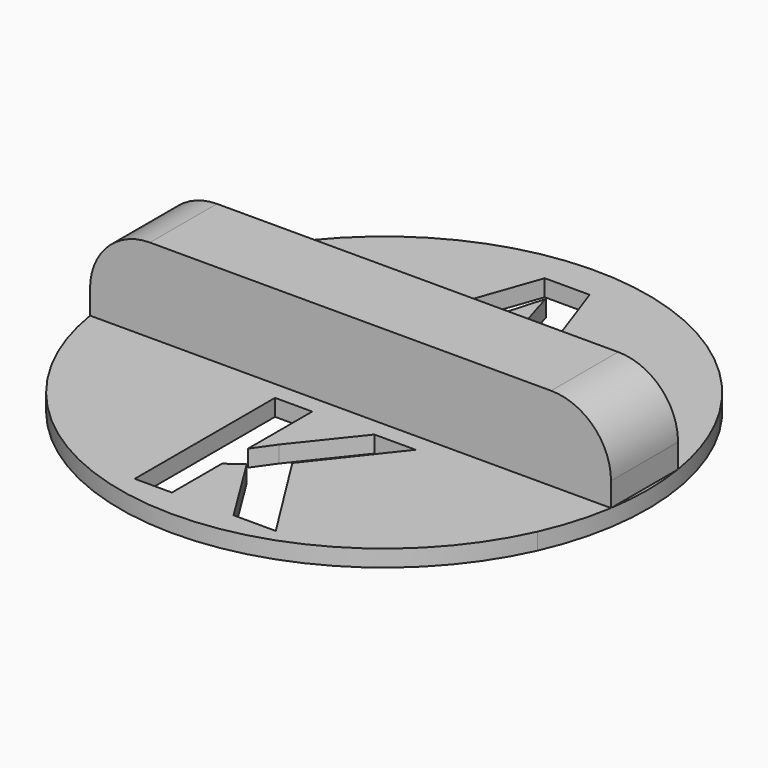
from build123d import *

# Parameters (mm, degrees)
F0_R          = 22.05
F1_DEPTH      = 1.4
F2_W          = 46.8786589982
F2_H          = 7
F3_DEPTH      = 7
F5_DEPTH      = 25
F7_DEPTH      = 25
F8_TEXT_SIZE  = 20.2705436904
F9_DEPTH      = 5
F10_TEXT_SIZE = 20.5177373977
F11_DEPTH     = 5


# Not quite as in the source:
# - Text() gives the source's letters only with a copy of the font that has no kerning and outlines rounded to 1/6400 em; it was checked with that copy


with BuildPart() as f1:
    # F0 (on Top) → F1 (new body)
    with BuildSketch(Plane.XY):
        Circle(F0_R)
    extrude(amount=F1_DEPTH)

    # F2 (on face) → F3 (join)
    with BuildSketch(Plane.XY.offset(1.4)):
        with Locations((0.6869044155, 0)):
            Rectangle(F2_W, F2_H)
    extrude(amount=F3_DEPTH)

    # F4 (on face) → F5 (cut)
    with BuildSketch(Plane.XY.offset(8.4)):
        with BuildLine():
            ThreePointArc((-20.2244413299, -8.784900278), (-22.0433329653, 0.1174414881), (-20.1296882775, 8.9998972133))
            Line((-20.1296882775, 8.9998972133), (-25.9023997933, 9.5238303766))
            Line((-25.9023997933, 9.5238303766), (-31.1410278082, -2.8289805632))
            Line((-31.1410278082, -2.8289805632), (-22.4099829793, -9.3610957265))
            Line((-22.4099829793, -9.3610957265), (-20.2244413299, -8.784900278))
        make_face()
        with BuildLine():
            Line((25.7077720016, 10.687969625), (18.850679885, 11.4391594041))
            ThreePointArc((18.850679885, 11.4391594041), (21.982729234, 1.3208352243), (20.0847610929, -9.0997182286))
            Line((20.0847610929, -9.0997182286), (27.3893084377, -8.0676069483))
            Line((27.3893084377, -8.0676069483), (31.0110747814, 2.2802972235))
            Line((31.0110747814, 2.2802972235), (25.7077720016, 10.687969625))
        make_face()
    extrude(amount=-F5_DEPTH, mode=Mode.SUBTRACT)

    # F6 (on face) → F7 (cut)
    with BuildSketch(Plane.XZ.offset(3.5)):
        with BuildLine():
            Line((-21.7650406008, 1.4), (-21.7650406008, 3.4))
            ThreePointArc((-21.7650406008, 3.4), (-20.3005745067, 6.9355339059), (-16.7650406008, 8.4))
            Line((-16.7650406008, 8.4), (-18.4185161579, 12.5083358405))
            Line((-18.4185161579, 12.5083358405), (-23.9234212786, 13.1551828235))
            Line((-23.9234212786, 13.1551828235), (-25.3046993166, 1.4))
            Line((-25.3046993166, 1.4), (-21.7650406008, 1.4))
        make_face()
        with BuildLine():
            ThreePointArc((16.7482826126, 8.4), (20.2838165185, 6.9355339059), (21.7482826126, 3.4))
            Line((21.7482826126, 3.4), (21.7482826126, 1.4))
            Line((21.7482826126, 1.4), (24.0328777581, 1.4))
            Line((24.0328777581, 1.4), (25.5436524749, 1.8891216023))
            Line((25.5436524749, 1.8891216023), (26.36378631, 8.6660245433))
            Line((26.36378631, 8.6660245433), (17.9466158152, 11.6875739768))
            Line((17.9466158152, 11.6875739768), (16.7482826126, 8.4))
        make_face()
    extrude(amount=-F7_DEPTH, mode=Mode.SUBTRACT)

    # F8 (on face) → F9 (cut)
    with BuildSketch(Plane.XY.offset(1.4)):
        with Locations((-7.0194806322, 4.621066153)):
            Text('A', F8_TEXT_SIZE, font='Open Sans', font_style=FontStyle.BOLD, text_align=(TextAlign.LEFT, TextAlign.BOTTOM))
    extrude(amount=-F9_DEPTH, mode=Mode.SUBTRACT)

    # F10 (on face) → F11 (cut)
    with BuildSketch(Plane.XY.offset(1.4)):
        with Locations((-6.9334963337, -19.6795873344)):
            Text('K', F10_TEXT_SIZE, font='Open Sans', font_style=FontStyle.BOLD, text_align=(TextAlign.LEFT, TextAlign.BOTTOM))
    extrude(amount=-F11_DEPTH, mode=Mode.SUBTRACT)


solid = f1.part
